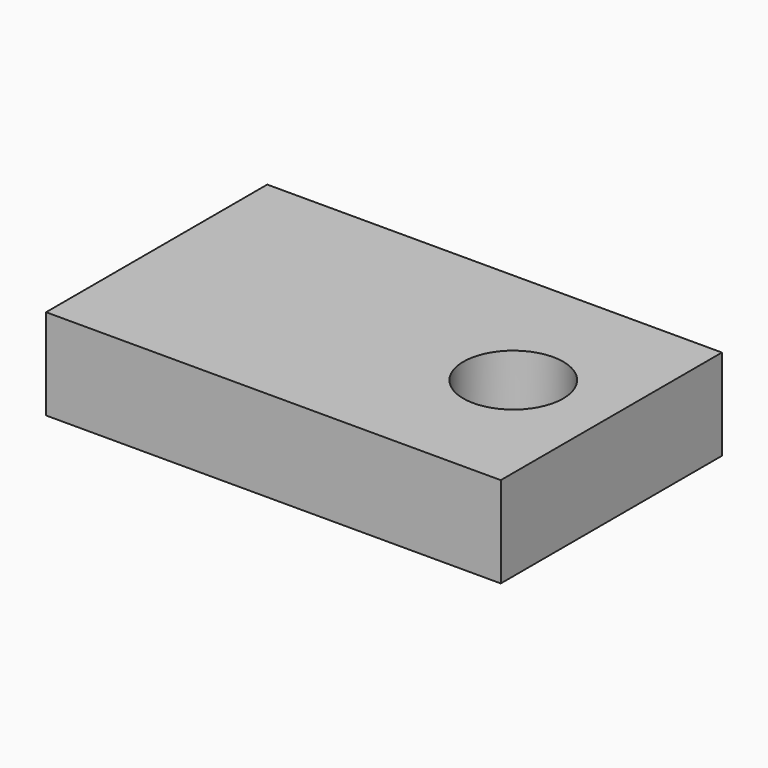
from build123d import *

# Parameters (mm, degrees)
F0_W     = 127
F0_H     = 77.2119465919
F0_R     = 13.9398216292
F1_DEPTH = 25.4


# Not quite as in the source:
# - the program builds the solid bodies; features that only make, move or delete a surface that nothing else refers to are left out


with BuildPart() as f1:
    # F0 (on Top) → F1 (new body)
    with BuildSketch(Plane.XY):
        Rectangle(F0_W, F0_H)
        with Locations((36.1109643691, 0)):
            Circle(F0_R, mode=Mode.SUBTRACT)
    extrude(amount=F1_DEPTH)


solid = f1.part
